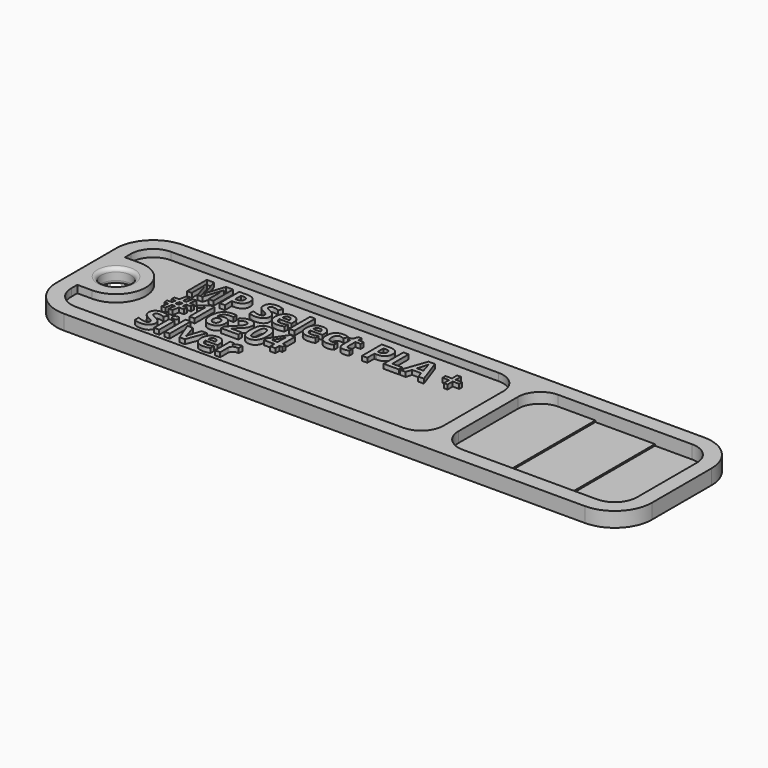
from build123d import *

# Parameters (mm, degrees)
F1_DEPTH      = 2
F3_DEPTH      = 1
F4_R          = 2
F5_DEPTH      = 2.001
F6_R          = 0.5
F7_DEPTH      = 0.4
F9_DEPTH      = 0.2
F11_DEPTH     = 0.2
F12_TEXT_SIZE = 4.6296296296
F13_DEPTH     = 0.6


# Not quite as in the source:
# - Text() gives the source's letters only with a copy of the font that has no kerning and outlines rounded to 1/6400 em; it was checked with that copy


with BuildPart() as f1:
    # F0 (on Top) → F1 (new body)
    with BuildSketch(Plane.XY):
        with BuildLine():
            ThreePointArc((40, 5), (38.5355339059, 8.5355339059), (35, 10))
            Line((35, 10), (-35, 10))
            ThreePointArc((-35, 10), (-38.5355339059, 8.5355339059), (-40, 5))
            Line((-40, 5), (-40, -5))
            ThreePointArc((-40, -5), (-38.5355339059, -8.5355339059), (-35, -10))
            Line((-35, -10), (35, -10))
            ThreePointArc((35, -10), (38.5355339059, -8.5355339059), (40, -5))
            Line((40, -5), (40, 5))
        make_face()
    extrude(amount=F1_DEPTH)

    # F2 (on face) → F3 (cut)
    with BuildSketch(Plane.XY.offset(2)):
        with BuildLine():
            ThreePointArc((35, -8), (37.1213203436, -7.1213203436), (38, -5))
            Line((38, -5), (38, 5))
            ThreePointArc((38, 5), (37.1213203436, 7.1213203436), (35, 8))
            Line((35, 8), (17, 8))
            ThreePointArc((17, 8), (14.8786796564, 7.1213203436), (14, 5))
            Line((14, 5), (14, -5))
            ThreePointArc((14, -5), (14.8786796564, -7.1213203436), (17, -8))
            Line((17, -8), (35, -8))
        make_face()
        with BuildLine():
            ThreePointArc((-38, -5), (-37.1213203436, -7.1213203436), (-35, -8))
            Line((-35, -8), (9, -8))
            ThreePointArc((9, -8), (11.1213203436, -7.1213203436), (12, -5))
            Line((12, -5), (12, 5))
            ThreePointArc((12, 5), (11.1213203436, 7.1213203436), (9, 8))
            Line((9, 8), (-35, 8))
            ThreePointArc((-35, 8), (-37.1213203436, 7.1213203436), (-38, 5))
            Line((-38, 5), (-38, 4))
            Line((-38, 4), (-36, 4))
            ThreePointArc((-36, 4), (-32, 0), (-36, -4))
            Line((-36, -4), (-38, -4))
            Line((-38, -4), (-38, -5))
        make_face()
    extrude(amount=-F3_DEPTH, mode=Mode.SUBTRACT)

    # F4 (on face) → F5 (cut, through all)
    with BuildSketch(Plane.XY.offset(2)):
        with Locations((-36, 0)):
            Circle(F4_R)
    extrude(amount=-F5_DEPTH, mode=Mode.SUBTRACT)

    # F6
    f6_edges = [f1.edges().sort_by_distance(p)[0] for p in [
        (-38, 0, 2),
        (-38, 0, 0),
    ]]
    fillet(f6_edges, radius=F6_R)

    # F7 (cut): a face of the model
    f7_faces = [f1.faces().sort_by_distance(p)[0] for p in [
        (26, 0, 1),
    ]]
    extrude(f7_faces, amount=-F7_DEPTH, mode=Mode.SUBTRACT)

    # F8 (on face) → F9 (cut)
    with BuildSketch(Plane.XY.offset(0.6)):
        with BuildLine():
            Line((22, -8), (35, -8))
            ThreePointArc((35, -8), (37.1213203436, -7.1213203436), (38, -5))
            Line((38, -5), (38, 5))
            ThreePointArc((38, 5), (37.1213203436, 7.1213203436), (35, 8))
            Line((35, 8), (22, 8))
            Line((22, 8), (22, -8))
        make_face()
    extrude(amount=-F9_DEPTH, mode=Mode.SUBTRACT)

    # F10 (on face) → F11 (cut)
    with BuildSketch(Plane.XY.offset(0.4)):
        with BuildLine():
            ThreePointArc((38, 5), (37.1213203436, 7.1213203436), (35, 8))
            Line((35, 8), (30, 8))
            Line((30, 8), (30, -8))
            Line((30, -8), (35, -8))
            ThreePointArc((35, -8), (37.1213203436, -7.1213203436), (38, -5))
            Line((38, -5), (38, 5))
        make_face()
    extrude(amount=-F11_DEPTH, mode=Mode.SUBTRACT)

    # F12 (on face) → F13 (join)
    with BuildSketch(Plane.XY.offset(1)):
        with Locations((-29, 2.6666666667)):
            Text('MP Select PLA +', F12_TEXT_SIZE, font='Open Sans', font_style=FontStyle.BOLD, text_align=(TextAlign.LEFT, TextAlign.BOTTOM))
        with Locations((-29, -1.6666666667)):
            Text('#16204', F12_TEXT_SIZE, font='Open Sans', font_style=FontStyle.BOLD, text_align=(TextAlign.LEFT, TextAlign.BOTTOM))
        with Locations((-29, -6)):
            Text('Silver', F12_TEXT_SIZE, font='Open Sans', font_style=FontStyle.BOLD, text_align=(TextAlign.LEFT, TextAlign.BOTTOM))
    extrude(amount=F13_DEPTH)


solid = f1.part
